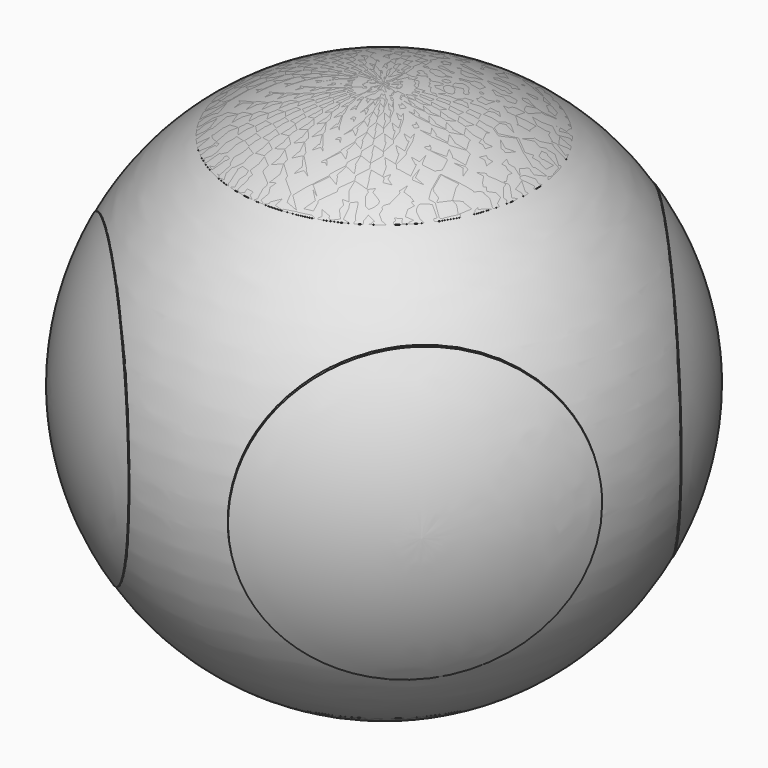
from build123d import *

# Parameters (mm, degrees)
F2_R     = 140
F3_DEPTH = 251.4968632571
F6_ANGLE = 90
F7_ANGLE = 90
F9_ANGLE = 45


with BuildPart() as f1:
    # F0 (on Right) → F1 (revolve)
    with BuildSketch(Plane.YZ):
        with BuildLine():
            ThreePointArc((1.4425029791, 243.5752286367), (172.7459651839, 171.7259570738), (243.5795, 0))
            ThreePointArc((243.5795, 0), (172.7459651839, -171.7259570738), (1.4425029791, -243.5752286367))
            Line((1.4425029791, -243.5752286367), (1.4425029791, -251.4958631571))
            ThreePointArc((1.4425029791, -251.4958631571), (178.3466280859, -177.3266202531), (251.5, 0))
            ThreePointArc((251.5, 0), (178.3466280859, 177.3266202531), (1.4425029791, 251.4958631571))
            Line((1.4425029791, 251.4958631571), (1.4425029791, 243.5752286367))
        make_face()
    revolve(axis=Axis((0, 1.4425029791, 80.1349282265), (0, 0, 1)))

    # F2 (on Top) → F3 (intersect, through all)
    with BuildSketch(Plane.XY):
        Circle(F2_R)
    extrude(amount=-F3_DEPTH, mode=Mode.INTERSECT)


with BuildPart() as f4_1:
    # F4: instance of F1
    add(f1.part.mirror(Plane.XY))


with BuildPart() as f5_1:
    # F5: instance of F4_1
    add(f4_1.part.mirror(Plane.XY))


with BuildPart() as f5_2:
    # F5: instance of F1
    add(f1.part.mirror(Plane.XY))


with BuildPart() as f6_1:
    # F6: copy of F5_2
    add(f5_2.part.rotate(Axis((0, -1.1176131666, 0), (0, 1, 0)), F6_ANGLE))


with BuildPart() as f6_2:
    # F6: copy of F5_1
    add(f5_1.part.rotate(Axis((0, -1.1176131666, 0), (0, 1, 0)), F6_ANGLE))


with BuildPart() as f4_1_1:
    # F7: moved
    add(f4_1.part.rotate(Axis((1.5088543296, 0, 0), (1, 0, 0)), F7_ANGLE))


with BuildPart() as f5_1_1:
    # F7: moved
    add(f5_1.part.rotate(Axis((1.5088543296, 0, 0), (1, 0, 0)), F7_ANGLE))


with BuildPart() as f8:
    # F0 (on Right) → F8 (revolve)
    with BuildSketch(Plane.YZ):
        with BuildLine():
            ThreePointArc((1.4425029791, 243.5752286367), (172.7459651839, 171.7259570738), (243.5795, 0))
            ThreePointArc((243.5795, 0), (172.7459651839, -171.7259570738), (1.4425029791, -243.5752286367))
            Line((1.4425029791, -243.5752286367), (1.4425029791, -251.4958631571))
            ThreePointArc((1.4425029791, -251.4958631571), (178.3466280859, -177.3266202531), (251.5, 0))
            ThreePointArc((251.5, 0), (178.3466280859, 177.3266202531), (1.4425029791, 251.4958631571))
            Line((1.4425029791, 251.4958631571), (1.4425029791, 243.5752286367))
        make_face()
    revolve(axis=Axis((0, 1.4425029791, -56.8897657667), (0, 0, -1)))


with BuildPart() as f6_1_1:
    # F9: moved
    add(f6_1.part.rotate(Axis((0, 1.4425029791, 80.1349282265), (0, 0, 1)), F9_ANGLE))


with BuildPart() as f6_2_1:
    # F9: moved
    add(f6_2.part.rotate(Axis((0, 1.4425029791, 80.1349282265), (0, 0, 1)), F9_ANGLE))


with BuildPart() as f5_1_2:
    # F9: moved
    add(f5_1_1.part.rotate(Axis((0, 1.4425029791, 80.1349282265), (0, 0, 1)), F9_ANGLE))


with BuildPart() as f5_2_1:
    # F9: moved
    add(f5_2.part.rotate(Axis((0, 1.4425029791, 80.1349282265), (0, 0, 1)), F9_ANGLE))


with BuildPart() as f4_1_2:
    # F9: moved
    add(f4_1_1.part.rotate(Axis((0, 1.4425029791, 80.1349282265), (0, 0, 1)), F9_ANGLE))


with BuildPart() as f1_1:
    # F9: moved
    add(f1.part.rotate(Axis((0, 1.4425029791, 80.1349282265), (0, 0, 1)), F9_ANGLE))


solid = Compound([f8.part, f6_1_1.part, f6_2_1.part, f5_1_2.part, f5_2_1.part, f4_1_2.part, f1_1.part])
